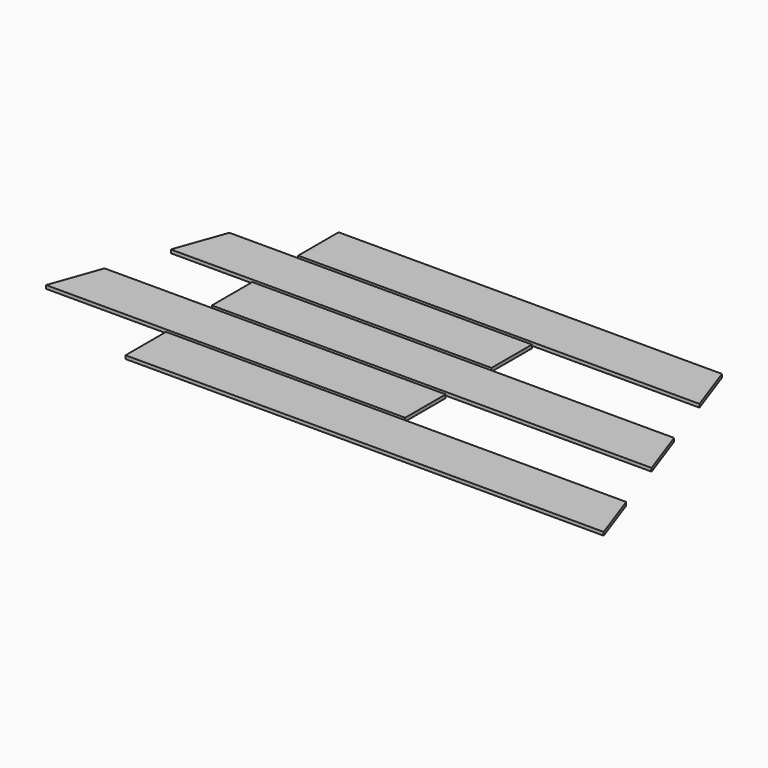
from build123d import *

# Parameters (mm, degrees)
F3_DEPTH = 2


# Not quite as in the source:
# - the program builds the solid bodies; features that only make, move or delete a surface that nothing else refers to are left out


with BuildPart() as f3:
    # F2 (on Top) → F3 (new body)
    with BuildSketch(Plane.XY):
        Polygon((-99.7756651271, -235.4982528798), (183.9081217199, -235.4982528798), (173.2191097174, -205.4982528798), (-99.7756651271, -205.4982528798), align=None)
    extrude(amount=F3_DEPTH)


with BuildPart() as f3b:
    # F2 (on Top) → F3, piece 2 (new body)
    with BuildSketch(Plane.XY):
        Polygon((-161.8174969148, -173.4982528798), (-172.5065089173, -203.4982528798), (40.5311334112, -203.4982528798), (40.5311334112, -173.4982528798), align=None)
    extrude(amount=F3_DEPTH)


with BuildPart() as f3c:
    # F2 (on Top) → F3, piece 3 (new body)
    with BuildSketch(Plane.XY):
        Polygon((-99.7756651271, -141.4982528798), (-99.7756651271, -171.4982528798), (161.1048961146, -171.4982528798), (150.4158841121, -141.4982528798), align=None)
    extrude(amount=F3_DEPTH)


with BuildPart() as f3d:
    # F2 (on Top) → F3, piece 4 (new body)
    with BuildSketch(Plane.XY):
        Polygon((-139.0142713095, -109.4982528798), (-149.703283312, -139.4982528798), (40.5311334112, -139.4982528798), (40.5311334112, -109.4982528798), align=None)
    extrude(amount=F3_DEPTH)


with BuildPart() as f3e:
    # F2 (on Top) → F3, piece 5 (new body)
    with BuildSketch(Plane.XY):
        Polygon((-99.7756651271, -107.4982528798), (138.3016705093, -107.4982528798), (127.6126585068, -77.4982528798), (-99.7756651271, -77.4982528798), align=None)
    extrude(amount=F3_DEPTH)


solid = Compound([f3.part, f3b.part, f3c.part, f3d.part, f3e.part])
